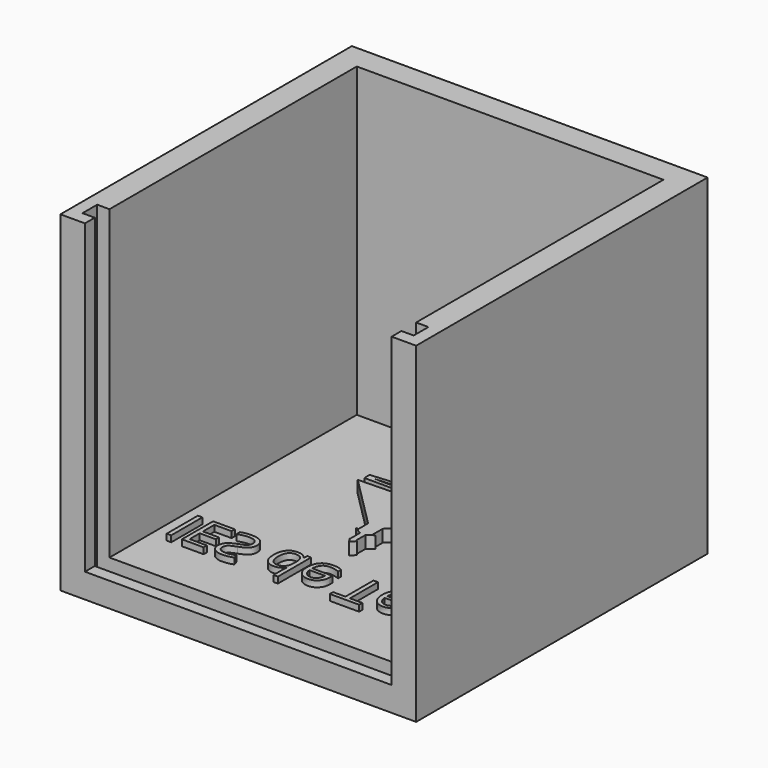
from build123d import *

# Parameters (mm, degrees)
F1_DEPTH     = 59.4
F2_W         = 58
F2_H         = 54
F3_DEPTH     = 4
F4_W         = 2
F4_H         = 3
F4_W_2       = 50
F5_DEPTH     = 52
F7_TEXT_SIZE = 8.9057558507
F8_DEPTH     = 3
F9_W         = 0.8984375745
F9_H         = 1.9921846688
F10_DEPTH    = 4


# Not quite as in the source:
# - Text() gives the source's letters only with a copy of the font that has no kerning and outlines rounded to 1/6400 em; it was checked with that copy


with BuildPart() as f1:
    # F0 (on Front) → F1 (new body)
    with BuildSketch(Plane.XZ):
        Polygon((0, 54), (0, 0), (58, 0), (58, 54), (54, 54), (54, 4), (4, 4), (4, 54), align=None)
    extrude(amount=F1_DEPTH)

    # F2 (on face) → F3 (join)
    with BuildSketch(Plane.XZ):
        with Locations((29, 27)):
            Rectangle(F2_W, F2_H)
    extrude(amount=F3_DEPTH)

    # F4 (on face) → F5 (cut)
    with BuildSketch(Plane.XY.offset(54)):
        with Locations((3, -55.9)):
            Rectangle(F4_W, F4_H)
        with Locations((29, -55.9)):
            Rectangle(F4_W_2, F4_H)
        with Locations((55, -55.9)):
            Rectangle(F4_W, F4_H)
    extrude(amount=-F5_DEPTH, mode=Mode.SUBTRACT)

    # F7 (on offset) → F8 (join)
    with BuildSketch(Plane(origin=(0, 0, 2), x_dir=(1, 0, 0), z_dir=(0, 0, -1))):
        with Locations((5.8981006123, 39.8505934059)):
            Text('IES de Teis', F7_TEXT_SIZE, font='Open Sans', text_align=(TextAlign.LEFT, TextAlign.BOTTOM))
    extrude(amount=-F8_DEPTH)

    # F9 (on offset) → F10 (join)
    with BuildSketch(Plane(origin=(0, 0, 2), x_dir=(1, 0, 0), z_dir=(0, 0, -1))):
        Polygon((28.1812131841, 34.163199014), (27.4976205517, 34.963979966), (26.9898076046, 34.163199014), (27.0679325301, 34.163199014), (27.9663701046, 34.163199014), align=None)
        with Locations((27.5171513174, 33.1671066796)):
            Rectangle(F9_W, F9_H)
        Polygon((27.9663701046, 32.1710143452), (27.0679325301, 32.1710143452), (25.8374635566, 31.4483564561), (26.2280881841, 31.4483564561), (26.2280881841, 29.475699759), (28.6109012056, 29.475699759), (28.6109012056, 31.4678881531), (29.0015258331, 31.4678881531), align=None)
        Polygon((28.6109012056, 29.475699759), (26.2280881841, 29.475699759), (17.6929302949, 20.9210101729), (35.8179334987, 20.4131990885), (36.7554326046, 21.3506981944), align=None)
        Polygon((36.4535443921, 19.9894063388), (18.055106743, 19.9894063388), (18.0194110114, 19.4481533235), (18.055106743, 18.8956573819), (33.4189922925, 17.7087680147), (20.457345822, 17.0229088492), (20.476981296, 16.5128443604), (20.457345822, 15.8120069035), (27.5472663167, 15.6133674785), (25.4569606755, 14.9695179735), (25.8285452116, 14.5987818231), (28.6109012056, 15.5835674514), (28.5905295184, 16.1127563185), (22.0689556139, 16.434342345), (34.8454470071, 17.0659737017), (35.3388032839, 17.5604589658), (35.3597954351, 18.3097195094), (19.1819940886, 19.3718272251), (36.981378371, 19.4627774876), align=None)
    extrude(amount=-F10_DEPTH)


solid = f1.part
